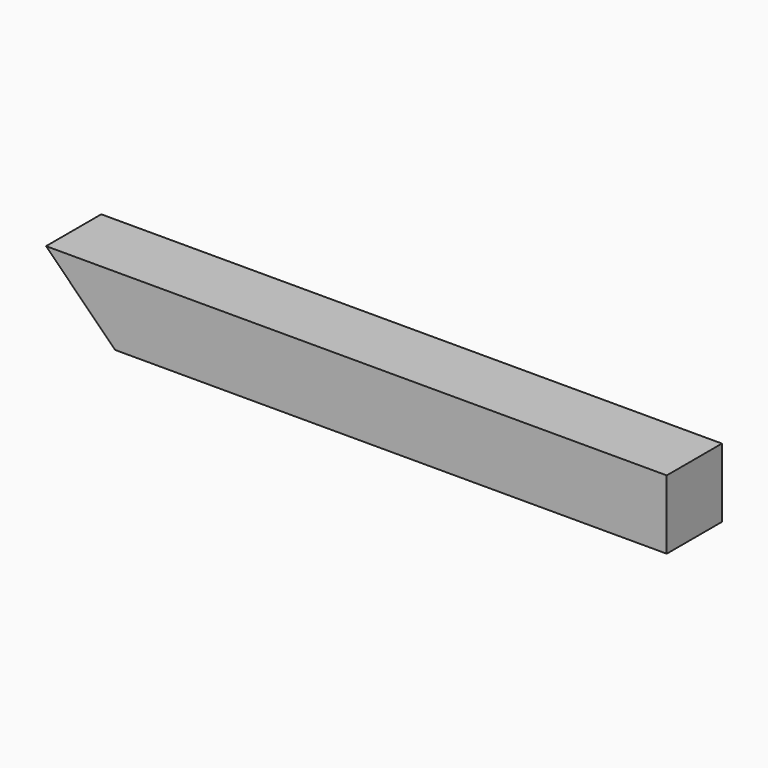
from build123d import *

# Parameters (mm, degrees)
F0_W     = 215.9
F0_H     = 25.4
F1_DEPTH = 25.4
F2_DEPTH = 12.7
F3_SIZE2 = 25.39999
F3_SIZE  = 25.39999


# Not quite as in the source:
# - a fillet or chamfer is up to 0.001 mm smaller than in the source, because OpenCascade refuses the exact size


with BuildPart() as f1:
    # F0 (on Front) → F1 (new body)
    with BuildSketch(Plane.XZ):
        with Locations((-71.4832603614, 24.0690046921)):
            Rectangle(F0_W, F0_H)
    extrude(amount=-F1_DEPTH)

    # F2 (add): a face of the model
    f2_faces = [f1.faces().sort_by_distance(p)[0] for p in [
        (36.4667396386, 12.7, 24.0690046921),
    ]]
    extrude(f2_faces, amount=F2_DEPTH)

    # F3 (size 25.4 and 25.4 in the source; OpenCascade refuses exactly that, so slightly less here)
    f3_edges = [f1.edges().sort_by_distance(p)[0] for p in [
        (-179.43326, 12.7, 11.369005),
    ]]
    chamfer(f3_edges, length=F3_SIZE, length2=F3_SIZE2)


solid = f1.part
